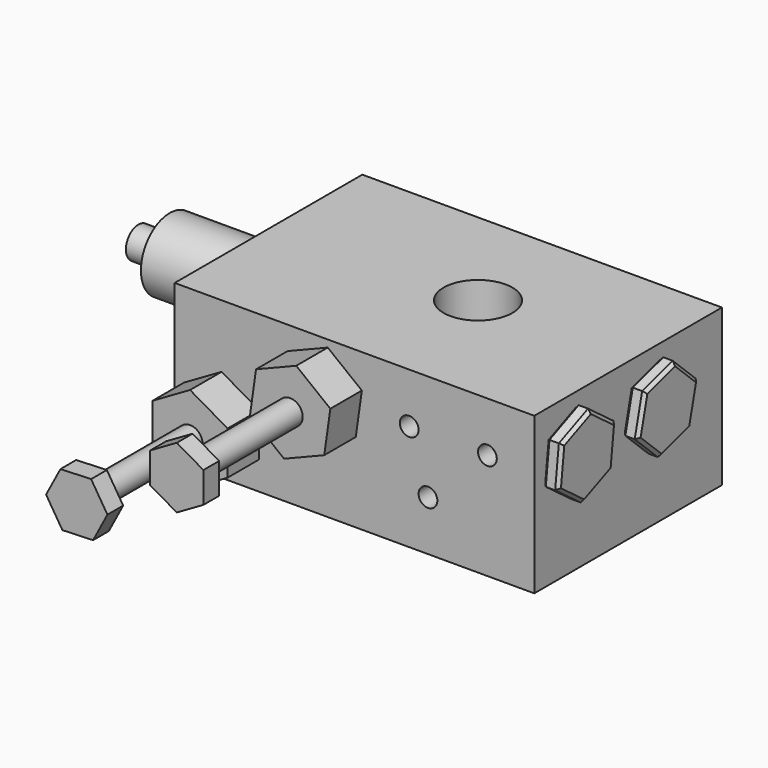
from build123d import *

# Parameters (mm, degrees)
F0_W            = 115
F0_H            = 75
F1_DEPTH        = 50
F3_D            = 5
F3_DEPTH        = 35
F3_TIP          = 1.5021515476
F5_D            = 13
F5_DEPTH        = 27
F5_CBORE_D      = 19
F5_CBORE_DEPTH  = 20
F5_TIP          = 3.9055940237
F7_D            = 6
F7_DEPTH        = 62
F7_TIP          = 1.8025818571
F9_D            = 6
F9_DEPTH        = 86
F9_TIP          = 1.8025818571
F10_D           = 13
F10_DEPTH       = 30
F10_CBORE_D     = 19
F10_CBORE_DEPTH = 22
F10_TIP         = 3.9055940237
F11_D           = 6
F11_DEPTH       = 8
F11_START       = 32.1030122
F11_TIP         = 1.8025818571
F12_D           = 6
F12_DEPTH       = 5
F12_START       = 29.1030122
F12_TIP         = 1.8025818571
F13_D           = 6
F13_DEPTH       = 16
F13_TIP         = 1.8025818571
F14_D           = 6
F14_DEPTH       = 30
F14_START       = 29.1030122
F14_TIP         = 1.8025818571
F15_D           = 6
F15_DEPTH       = 50
F15_TIP         = 1.8025818571
F16_D           = 6
F16_DEPTH       = 34
F16_TIP         = 1.8025818571
F17_D           = 13
F17_DEPTH       = 30
F17_CBORE_D     = 19
F17_CBORE_DEPTH = 22
F17_TIP         = 3.9055940237
F18_D           = 6
F18_DEPTH       = 15
F18_START       = 32.1030122
F18_TIP         = 1.8025818571
F19_D           = 6
F19_DEPTH       = 35
F19_TIP         = 1.8025818571
F20_D           = 6
F20_DEPTH       = 6
F20_START       = 32.1030122
F20_TIP         = 1.8025818571
F22_D           = 5
F22_DEPTH       = 15
F22_TIP         = 1.5021515476
F23_D           = 22
F24_R           = 11.5
F25_DEPTH       = 26
F27_D           = 13
F27_DEPTH       = 30
F27_CBORE_D     = 19
F27_CBORE_DEPTH = 22
F27_TIP         = 3.9055940237
F28_D           = 6
F28_DEPTH       = 85
F28_TIP         = 1.8025818571
F29_DEPTH       = 5
F30_SIZE        = 1
F30_2_SIZE      = 1
F26_R           = 5
F31_DEPTH       = 12
F8_R            = 11.5
F32_DEPTH       = 30
F33_R           = 5
F34_DEPTH       = 10
F35_D           = 6
F35_DEPTH       = 18
F35_TIP         = 1.8025818571
F37_DEPTH       = 12.6
F38_R           = 4
F39_DEPTH       = 39
F40_R           = 4
F41_DEPTH       = 6.3
F42_R           = 4
F43_DEPTH       = 39
F44_R           = 4
F45_DEPTH       = 6.3
F46_D           = 5
F46_DEPTH       = 6
F46_TIP         = 1.5021515476


# Not quite as in the source:
# - a feature names something its author has since deleted; it is built from what else it names


with BuildPart() as f1:
    # F0 (on Top) → F1 (new body)
    with BuildSketch(Plane.XY):
        with Locations((-7.5, -2.5)):
            Rectangle(F0_W, F0_H)
    extrude(amount=F1_DEPTH)

    # F3
    with Locations(Plane(origin=(0, 0, 0), x_dir=(1, 0, 0), z_dir=(0, 0, -1))):
        with Locations((16, -7.32)):
            Hole(F3_D / 2, depth=F3_DEPTH)
            with Locations((0, 0, -(F3_DEPTH + F3_TIP / 2))):  # 118° drill point
                Cone(0, F3_D / 2, F3_TIP, mode=Mode.SUBTRACT)

    # F5
    with Locations(Plane.YZ.offset(50)):
        with Locations((7.32, 34), (-25, 34)):
            CounterBoreHole(F5_D / 2, F5_CBORE_D / 2, F5_CBORE_DEPTH, depth=F5_DEPTH)
            with Locations((0, 0, -(F5_DEPTH + F5_TIP / 2))):  # 118° drill point
                Cone(0, F5_D / 2, F5_TIP, mode=Mode.SUBTRACT)

    # F7
    with Locations(Plane.XZ.offset(40)):
        with Locations((16, 16)):
            Hole(F7_D / 2, depth=F7_DEPTH)
            with Locations((0, 0, -(F7_DEPTH + F7_TIP / 2))):  # 118° drill point
                Cone(0, F7_D / 2, F7_TIP, mode=Mode.SUBTRACT)

    # F9
    with Locations(Plane(origin=(-65, 0, 0), x_dir=(0, -1, 0), z_dir=(-1, 0, 0))):
        with Locations((25, 16)):
            Hole(F9_D / 2, depth=F9_DEPTH)
            with Locations((0, 0, -(F9_DEPTH + F9_TIP / 2))):  # 118° drill point
                Cone(0, F9_D / 2, F9_TIP, mode=Mode.SUBTRACT)

    # F10
    with Locations(Plane.XZ.offset(40)):
        with Locations((-50, 16), (-18, 34)):
            CounterBoreHole(F10_D / 2, F10_CBORE_D / 2, F10_CBORE_DEPTH, depth=F10_DEPTH)
            with Locations((0, 0, -(F10_DEPTH + F10_TIP / 2))):  # 118° drill point
                Cone(0, F10_D / 2, F10_TIP, mode=Mode.SUBTRACT)

    # F11
    # its depths count from where the whole tool has entered the part; down to there all is cleared
    with Locations(Plane.XZ.offset(40)):
        with Locations((-50, 16)):
            Hole(F11_D / 2, depth=F11_START)
    with Locations(Plane.XZ.offset(40).offset(-F11_START)):
        with Locations((-50, 16)):
            Hole(F11_D / 2, depth=F11_DEPTH)
            with Locations((0, 0, -(F11_DEPTH + F11_TIP / 2))):  # 118° drill point
                Cone(0, F11_D / 2, F11_TIP, mode=Mode.SUBTRACT)

    # F12
    # its depths count from where the whole tool has entered the part; down to there all is cleared
    with Locations(Plane.YZ.offset(50)):
        with Locations((7.32, 34)):
            Hole(F12_D / 2, depth=F12_START)
    with Locations(Plane.YZ.offset(50).offset(-F12_START)):
        with Locations((7.32, 34)):
            Hole(F12_D / 2, depth=F12_DEPTH)
            with Locations((0, 0, -(F12_DEPTH + F12_TIP / 2))):  # 118° drill point
                Cone(0, F12_D / 2, F12_TIP, mode=Mode.SUBTRACT)

    # F13
    with Locations(Plane.XZ.offset(40)):
        with Locations((10, 34)):
            Hole(F13_D / 2, depth=F13_DEPTH)
            with Locations((0, 0, -(F13_DEPTH + F13_TIP / 2))):  # 118° drill point
                Cone(0, F13_D / 2, F13_TIP, mode=Mode.SUBTRACT)

    # F14
    # its depths count from where the whole tool has entered the part; down to there all is cleared
    with Locations(Plane.YZ.offset(50).offset(-F14_START)):
        with Locations((-25, 34)):
            Hole(F14_D / 2, depth=F14_DEPTH)
            with Locations((0, 0, -(F14_DEPTH + F14_TIP / 2))):  # 118° drill point
                Cone(0, F14_D / 2, F14_TIP, mode=Mode.SUBTRACT)

    # F15
    with Locations(Plane.XZ.offset(40)):
        with Locations((35, 34)):
            Hole(F15_D / 2, depth=F15_DEPTH)
            with Locations((0, 0, -(F15_DEPTH + F15_TIP / 2))):  # 118° drill point
                Cone(0, F15_D / 2, F15_TIP, mode=Mode.SUBTRACT)

    # F16
    with Locations(Plane(origin=(0, 0, 0), x_dir=(1, 0, 0), z_dir=(0, 0, -1))):
        with Locations((35, 9)):
            Hole(F16_D / 2, depth=F16_DEPTH)
            with Locations((0, 0, -(F16_DEPTH + F16_TIP / 2))):  # 118° drill point
                Cone(0, F16_D / 2, F16_TIP, mode=Mode.SUBTRACT)

    # F17
    with Locations(Plane(origin=(-65, 0, 0), x_dir=(0, -1, 0), z_dir=(-1, 0, 0))):
        with Locations((4.5, 34)):
            CounterBoreHole(F17_D / 2, F17_CBORE_D / 2, F17_CBORE_DEPTH, depth=F17_DEPTH)
            with Locations((0, 0, -(F17_DEPTH + F17_TIP / 2))):  # 118° drill point
                Cone(0, F17_D / 2, F17_TIP, mode=Mode.SUBTRACT)

    # F18
    # its depths count from where the whole tool has entered the part; down to there all is cleared
    with Locations(Plane(origin=(-65, 0, 0), x_dir=(0, -1, 0), z_dir=(-1, 0, 0))):
        with Locations((4.5, 34)):
            Hole(F18_D / 2, depth=F18_START)
    with Locations(Plane(origin=(-65, 0, 0), x_dir=(0, -1, 0), z_dir=(-1, 0, 0)).offset(-F18_START)):
        with Locations((4.5, 34)):
            Hole(F18_D / 2, depth=F18_DEPTH)
            with Locations((0, 0, -(F18_DEPTH + F18_TIP / 2))):  # 118° drill point
                Cone(0, F18_D / 2, F18_TIP, mode=Mode.SUBTRACT)

    # F19
    with Locations(Plane(origin=(0, 0, 0), x_dir=(1, 0, 0), z_dir=(0, 0, -1))):
        with Locations((-50, 2)):
            Hole(F19_D / 2, depth=F19_DEPTH)
            with Locations((0, 0, -(F19_DEPTH + F19_TIP / 2))):  # 118° drill point
                Cone(0, F19_D / 2, F19_TIP, mode=Mode.SUBTRACT)

    # F20
    # its depths count from where the whole tool has entered the part; down to there all is cleared
    with Locations(Plane.XZ.offset(40)):
        with Locations((-18, 34)):
            Hole(F20_D / 2, depth=F20_START)
    with Locations(Plane.XZ.offset(40).offset(-F20_START)):
        with Locations((-18, 34)):
            Hole(F20_D / 2, depth=F20_DEPTH)
            with Locations((0, 0, -(F20_DEPTH + F20_TIP / 2))):  # 118° drill point
                Cone(0, F20_D / 2, F20_TIP, mode=Mode.SUBTRACT)

    # F22
    with Locations(Plane(origin=(0, 35, 0), x_dir=(-1, 0, 0), z_dir=(0, 1, 0))):
        with Locations((50, 35), (-35, 35)):
            Hole(F22_D / 2, depth=F22_DEPTH)
            with Locations((0, 0, -(F22_DEPTH + F22_TIP / 2))):  # 118° drill point
                Cone(0, F22_D / 2, F22_TIP, mode=Mode.SUBTRACT)

    # F23 (through all)
    with Locations(Plane(origin=(0, 0, 0), x_dir=(1, 0, 0), z_dir=(0, 0, -1))):
        with Locations((0, 0)):
            Hole(F23_D / 2)

    # F27
    with Locations(Plane(origin=(-65, 0, 0), x_dir=(0, -1, 0), z_dir=(-1, 0, 0))):
        with Locations((-20, 16)):
            CounterBoreHole(F27_D / 2, F27_CBORE_D / 2, F27_CBORE_DEPTH, depth=F27_DEPTH)
            with Locations((0, 0, -(F27_DEPTH + F27_TIP / 2))):  # 118° drill point
                Cone(0, F27_D / 2, F27_TIP, mode=Mode.SUBTRACT)

    # F28
    with Locations(Plane(origin=(-65, 0, 0), x_dir=(0, -1, 0), z_dir=(-1, 0, 0))):
        with Locations((-20, 16)):
            Hole(F28_D / 2, depth=F28_DEPTH)
            with Locations((0, 0, -(F28_DEPTH + F28_TIP / 2))):  # 118° drill point
                Cone(0, F28_D / 2, F28_TIP, mode=Mode.SUBTRACT)

    # F35
    with Locations(Plane(origin=(0, 0, 0), x_dir=(1, 0, 0), z_dir=(0, 0, -1))):
        with Locations((-50, -20)):
            Hole(F35_D / 2, depth=F35_DEPTH)
            with Locations((0, 0, -(F35_DEPTH + F35_TIP / 2))):  # 118° drill point
                Cone(0, F35_D / 2, F35_TIP, mode=Mode.SUBTRACT)

    # F46
    with Locations(Plane(origin=(0, 0, 0), x_dir=(1, 0, 0), z_dir=(0, 0, -1))):
        with Locations((-16, -22.32), (16, 7.68)):
            Hole(F46_D / 2, depth=F46_DEPTH)
            with Locations((0, 0, -(F46_DEPTH + F46_TIP / 2))):  # 118° drill point
                Cone(0, F46_D / 2, F46_TIP, mode=Mode.SUBTRACT)


with BuildPart() as f25:
    # F24 (on face) → F25 (new body)
    with BuildSketch(Plane(origin=(-65, 0, 0), x_dir=(0, -1, 0), z_dir=(-1, 0, 0))):
        with Locations((-20, 16)):
            Circle(F24_R)
    extrude(amount=F25_DEPTH)

    # F26 (on face) → F31 (join)
    with BuildSketch(Plane(origin=(-91, 0, 0), x_dir=(0, -1, 0), z_dir=(-1, 0, 0))):
        with Locations((-20, 16)):
            Circle(F26_R)
    extrude(amount=F31_DEPTH)


with BuildPart() as f29:
    # F4 (on face) → F29 (new body)
    with BuildSketch(Plane.YZ.offset(50)):
        Polygon((-23.5270221617, 46.6160084663), (-35.189294907, 41.5836404603), (-36.6622727453, 28.967631994), (-26.4729778383, 21.3839915337), (-14.810705093, 26.4163595397), (-13.3377272547, 39.032368006), align=None)
    extrude(amount=F29_DEPTH)

    # F30
    f30_edges = [f29.edges().sort_by_distance(p)[0] for p in [
        (50, -20.641841, 23.900176),
        (50, -31.567625, 25.175812),
        (50, -35.925784, 35.275636),
        (55, -31.567625, 25.175812),
        (55, -20.641841, 23.900176),
        (55, -14.074216, 32.724364),
        (55, -18.432375, 42.824188),
        (55, -29.358159, 44.099824),
        (55, -35.925784, 35.275636),
        (50, -29.358159, 44.099824),
        (50, -18.432375, 42.824188),
        (50, -14.074216, 32.724364),
    ]]
    chamfer(f30_edges, length=F30_SIZE)


with BuildPart() as f29b:
    # F4 (on face) → F29, piece 2 (new body)
    with BuildSketch(Plane.YZ.offset(50)):
        Polygon((10.3008178574, 46.3469857955), (-1.8823944304, 42.7549568863), (-4.8632122878, 30.4079710908), (4.3391821426, 21.6530142045), (16.5223944304, 25.2450431137), (19.5032122878, 37.5920289092), align=None)
    extrude(amount=F29_DEPTH)

    # F30#2
    f30_2_edges = [f29b.edges().sort_by_distance(p)[0] for p in [
        (55, -0.262015, 26.030493),
        (50, -0.262015, 26.030493),
        (55, 10.430788, 23.449029),
        (50, 10.430788, 23.449029),
        (55, 18.012803, 31.418536),
        (50, 18.012803, 31.418536),
        (55, 14.902015, 41.969507),
        (50, 14.902015, 41.969507),
        (55, -3.372803, 36.581464),
        (50, -3.372803, 36.581464),
        (50, 4.209212, 44.550971),
        (55, 4.209212, 44.550971),
    ]]
    chamfer(f30_2_edges, length=F30_2_SIZE)


with BuildPart() as f32:
    # F8 (on face) → F32 (new body)
    with BuildSketch(Plane(origin=(-65, 0, 0), x_dir=(0, -1, 0), z_dir=(-1, 0, 0))):
        with Locations((4.5, 34)):
            Circle(F8_R)
    extrude(amount=F32_DEPTH)

    # F33 (on face) → F34 (join)
    with BuildSketch(Plane(origin=(-95, 0, 0), x_dir=(0, -1, 0), z_dir=(-1, 0, 0))):
        with Locations((4.5, 34)):
            Circle(F33_R)
    extrude(amount=F34_DEPTH)


with BuildPart() as f37:
    # F36 (on face) → F37 (new body)
    with BuildSketch(Plane.XZ.offset(40)):
        Polygon((-38, 9.0717967697), (-38, 22.9282032303), (-50, 29.8564064606), (-62, 22.9282032303), (-62, 9.0717967697), (-50, 2.1435935394), align=None)
    extrude(amount=F37_DEPTH)

    # F38 (on face) → F39 (join)
    with BuildSketch(Plane.XZ.offset(52.6)):
        with Locations((-50, 16)):
            Circle(F38_R)
    extrude(amount=F39_DEPTH)

    # F40 (on face) → F41 (join)
    with BuildSketch(Plane.XZ.offset(91.6)):
        Polygon((-40.1919154978, 16.3671671712), (-45.4139338466, 24.6776339269), (-55.2220183487, 24.3104667558), (-59.8080845022, 15.6328328288), (-54.5860661534, 7.3223660731), (-44.7779816513, 7.6895332442), align=None)
        with Locations((-50, 16)):
            Circle(F40_R, mode=Mode.SUBTRACT)
        with Locations((-50, 16)):
            Circle(F40_R)
    extrude(amount=F41_DEPTH)


with BuildPart() as f37b:
    # F36 (on face) → F37, piece 2 (new body)
    with BuildSketch(Plane.XZ.offset(40)):
        Polygon((-7.0902049982, 25.4573790311), (-5.1469757251, 39.1768491372), (-16.056770727, 47.7194701061), (-28.9097950018, 42.5426209689), (-30.8530242749, 28.8231508628), (-19.943229273, 20.2805298939), align=None)
    extrude(amount=F37_DEPTH)

    # F42 (on face) → F43 (join)
    with BuildSketch(Plane.XZ.offset(52.6)):
        with Locations((-18, 34)):
            Circle(F42_R)
    extrude(amount=F43_DEPTH)

    # F44 (on face) → F45 (join)
    with BuildSketch(Plane.XZ.offset(91.6)):
        Polygon((-9.5, 29.0925227119), (-9.5, 38.9074772881), (-18, 43.8149545762), (-26.5, 38.9074772881), (-26.5, 29.0925227119), (-18, 24.1850454238), align=None)
        with Locations((-18, 34)):
            Circle(F44_R, mode=Mode.SUBTRACT)
        with Locations((-18, 34)):
            Circle(F44_R)
    extrude(amount=F45_DEPTH)


solid = Compound([f1.part, f25.part, f29.part, f29b.part, f32.part, f37.part, f37b.part])
